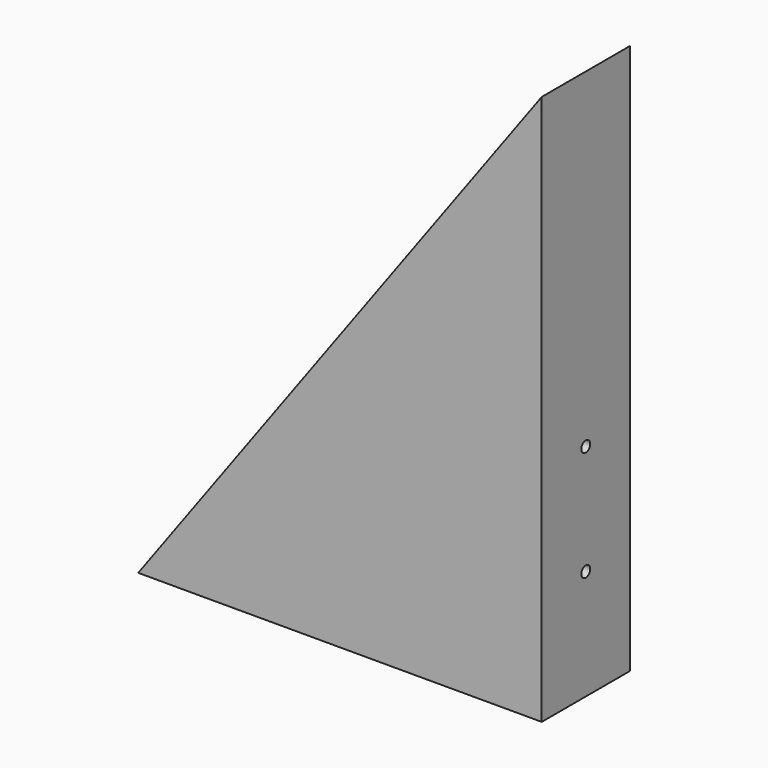
from build123d import *

# Parameters (mm, degrees)
F1_DEPTH = 30
F2_R     = 1.5
F3_DEPTH = 25


# Not quite as in the source:
# - a feature names something its author has since deleted; it is built from what else it names


with BuildPart() as f1:
    # F0 (on Front) → F1 (new body)
    with BuildSketch(Plane.XZ):
        Polygon((110, 150), (0, 0), (110, 0), align=None)
    extrude(amount=F1_DEPTH)

    # F2 (on face) → F3 (cut)
    with BuildSketch(Plane.YZ.offset(110)):
        with Locations((-15, 30)):
            Circle(F2_R)
        with Locations((-15, 60)):
            Circle(F2_R)
    extrude(amount=-F3_DEPTH, mode=Mode.SUBTRACT)


solid = f1.part
